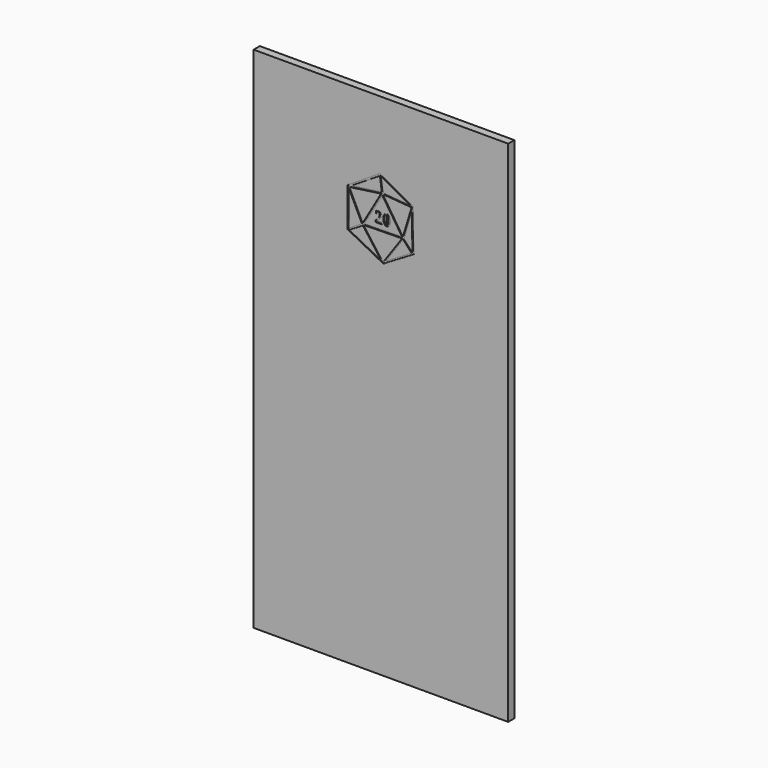
from build123d import *

# Parameters (mm, degrees)
F0_TEXT_SIZE = 10.5298538175
F1_DEPTH     = 4.5
F0_W         = 165
F0_H         = 330
F2_DEPTH     = 5


# Not quite as in the source:
# - Text() gives the source's letters only with a copy of the font that has no kerning and outlines rounded to 1/6400 em; it was checked with that copy


with BuildPart() as f1:
    # F0 (on Front) → F1 (new body)
    with BuildSketch(Plane.XZ):
        Polygon((-14.2118764941, 152.9690027237), (8.9000429127, 140.9807896144), (28.7076475199, 152.7439020574), (28.2208197919, 179.8401356328), (6.6943259021, 191.7312443256), (-14.2118764941, 178.4029453993), align=None)
        Polygon((-4.3210338262, 158.3704430342), (6.9607992757, 143.0644951761), (-13.3234340052, 152.9690027237), align=None, mode=Mode.SUBTRACT)
        Polygon((-5.0023751624, 159.2944927975), (-13.229465754, 154.1256457567), (-13.205724124, 176.2030571699), align=None, mode=Mode.SUBTRACT)
        Polygon((7.4572008215, 180.4599764734), (-4.2189589601, 160.2786725549), (-12.6338905555, 177.6233464479), align=None, mode=Mode.SUBTRACT)
        Polygon((7.8499403882, 181.5359219909), (-11.4866445672, 178.9970174432), (6.6943259021, 190.3372129676), align=None, mode=Mode.SUBTRACT)
        Polygon((21.0209441463, 159.2944927975), (8.9000429127, 142.0140191913), (-3.5439810615, 158.8966995478), align=None, mode=Mode.SUBTRACT)
        Polygon((27.1449846316, 152.9690027237), (10.6374726731, 143.0644951761), (21.7425262656, 158.8966995478), align=None, mode=Mode.SUBTRACT)
        Polygon((21.0209441463, 160.2786725549), (-3.3660947245, 159.8837599158), (8.2897230152, 179.6133667231), align=None, mode=Mode.SUBTRACT)
        Polygon((9.2267788116, 180.4651319981), (27.2039122048, 178.9970174432), (21.6317921941, 160.7204639738), align=None, mode=Mode.SUBTRACT)
        Polygon((27.7245932359, 153.8676992059), (22.3661095936, 159.7770527005), (27.3740378309, 176.2030571699), align=None, mode=Mode.SUBTRACT)
        Polygon((8.9000429127, 181.4443767071), (7.6089858178, 190.2102828026), (26.0070047419, 180.0473252917), align=None, mode=Mode.SUBTRACT)
        with Locations((3.2967818536, 163.0602906743)):
            Text('20', F0_TEXT_SIZE, font='Tinos', font_style=FontStyle.BOLD, text_align=(TextAlign.LEFT, TextAlign.BOTTOM))
    extrude(amount=F1_DEPTH)

    # F0 (on Front) → F2 (join)
    with BuildSketch(Plane.XZ):
        with Locations((7.302631028, 70.7766927429)):
            Rectangle(F0_W, F0_H)
        Polygon((28.7076475199, 152.7439020574), (8.9000429127, 140.9807896144), (-14.2118764941, 152.9690027237), (-14.2118764941, 178.4029453993), (6.6943259021, 191.7312443256), (28.2208197919, 179.8401356328), align=None, mode=Mode.SUBTRACT)
        Polygon((-13.3234340052, 152.9690027237), (6.9607992757, 143.0644951761), (-4.3210338262, 158.3704430342), align=None)
        Polygon((-13.205724124, 176.2030571699), (-13.229465754, 154.1256457567), (-5.0023751624, 159.2944927975), align=None)
        Polygon((-12.6338905555, 177.6233464479), (-4.2189589601, 160.2786725549), (7.4572008215, 180.4599764734), align=None)
        Polygon((6.6943259021, 190.3372129676), (-11.4866445672, 178.9970174432), (7.8499403882, 181.5359219909), align=None)
        Polygon((26.0070047419, 180.0473252917), (7.6089858178, 190.2102828026), (8.9000429127, 181.4443767071), align=None)
        Polygon((21.6317921941, 160.7204639738), (27.2039122048, 178.9970174432), (9.2267788116, 180.4651319981), align=None)
        Polygon((27.3740378309, 176.2030571699), (22.3661095936, 159.7770527005), (27.7245932359, 153.8676992059), align=None)
        Polygon((21.7425262656, 158.8966995478), (10.6374726731, 143.0644951761), (27.1449846316, 152.9690027237), align=None)
        Polygon((-3.5439810615, 158.8966995478), (8.9000429127, 142.0140191913), (21.0209441463, 159.2944927975), align=None)
        Polygon((8.2897230152, 179.6133667231), (-3.3660947245, 159.8837599158), (21.0209441463, 160.2786725549), align=None)
        with BuildLine():
            Line((8.1092541061, 164.2218651736), (8.1092541061, 163.0602906743))
            Line((8.1092541061, 163.0602906743), (3.7393647718, 163.0602906743))
            Line((3.7393647718, 163.0602906743), (3.7393647718, 164.0326568628))
            add(Edge.make_bspline(
                [(3.7393647718, 164.0326568628), (4.1819476901, 164.5048549949), (4.5570737323, 164.8799810372)],
                knots=[0, 0, 0, 1, 1, 1], degree=2))
            add(Edge.make_bspline(
                [(4.5570737323, 164.8799810372), (5.3797185618, 165.6927541287), (5.7597804731, 166.1583711022)],
                knots=[0, 0, 0, 1, 1, 1], degree=2))
            add(Edge.make_bspline(
                [(5.7597804731, 166.1583711022), (6.1398423843, 166.6239880757), (6.3175336674, 167.1225108424)],
                knots=[0, 0, 0, 1, 1, 1], degree=2))
            add(Edge.make_bspline(
                [(6.3175336674, 167.1225108424), (6.4952249506, 167.621033609), (6.4952249506, 168.2577607071)],
                knots=[0, 0, 0, 1, 1, 1], degree=2))
            add(Edge.make_bspline(
                [(6.4952249506, 168.2577607071), (6.4952249506, 168.8188044808), (6.2229295121, 169.1634926643)],
                knots=[0, 0, 0, 1, 1, 1], degree=2))
            add(Edge.make_bspline(
                [(6.2229295121, 169.1634926643), (5.9506340735, 169.5081808479), (5.4981794173, 169.5081808479)],
                knots=[0, 0, 0, 1, 1, 1], degree=2))
            add(Edge.make_bspline(
                [(5.4981794173, 169.5081808479), (5.1789932234, 169.5081808479), (4.9889622678, 169.4415466167)],
                knots=[0, 0, 0, 1, 1, 1], degree=2))
            add(Edge.make_bspline(
                [(4.9889622678, 169.4415466167), (4.7989313122, 169.3749123855), (4.6393382153, 169.2399986335)],
                knots=[0, 0, 0, 1, 1, 1], degree=2))
            Line((4.6393382153, 169.2399986335), (4.4172241113, 168.2429531001))
            Line((4.4172241113, 168.2429531001), (3.9697053241, 168.2429531001))
            Line((3.9697053241, 168.2429531001), (3.9697053241, 169.8109141451))
            add(Edge.make_bspline(
                [(3.9697053241, 169.8109141451), (4.3810277388, 169.903050366), (4.7750746122, 169.9680393076)],
                knots=[0, 0, 0, 1, 1, 1], degree=2))
            add(Edge.make_bspline(
                [(4.7750746122, 169.9680393076), (5.1691214855, 170.0330282491), (5.6314478797, 170.0330282491)],
                knots=[0, 0, 0, 1, 1, 1], degree=2))
            add(Edge.make_bspline(
                [(5.6314478797, 170.0330282491), (6.7666977444, 170.0330282491), (7.371341694, 169.5649433411)],
                knots=[0, 0, 0, 1, 1, 1], degree=2))
            add(Edge.make_bspline(
                [(7.371341694, 169.5649433411), (7.9759856437, 169.0968584331), (7.9759856437, 168.2330813622)],
                knots=[0, 0, 0, 1, 1, 1], degree=2))
            add(Edge.make_bspline(
                [(7.9759856437, 168.2330813622), (7.9759856437, 167.693426354), (7.795826426, 167.2533113702)],
                knots=[0, 0, 0, 1, 1, 1], degree=2))
            add(Edge.make_bspline(
                [(7.795826426, 167.2533113702), (7.6156672084, 166.8131963865), (7.2273788489, 166.3969381027)],
                knots=[0, 0, 0, 1, 1, 1], degree=2))
            add(Edge.make_bspline(
                [(7.2273788489, 166.3969381027), (6.8390904893, 165.980679819), (5.6824518591, 165.0395741341)],
                knots=[0, 0, 0, 1, 1, 1], degree=2))
            add(Edge.make_bspline(
                [(5.6824518591, 165.0395741341), (5.2398689408, 164.6792556988), (4.7265385672, 164.2218651736)],
                knots=[0, 0, 0, 1, 1, 1], degree=2))
            Line((4.7265385672, 164.2218651736), (8.1092541061, 164.2218651736))
        make_face(mode=Mode.SUBTRACT)
        with BuildLine():
            add(Edge.make_bspline(
                [(12.8600279964, 169.1659605988), (13.4251849943, 168.2692777347), (13.4251849943, 166.5367877238)],
                knots=[0, 0, 0, 1, 1, 1], degree=2))
            add(Edge.make_bspline(
                [(13.4251849943, 166.5367877238), (13.4251849943, 162.9566374258), (11.1629117132, 162.9566374258)],
                knots=[0, 0, 0, 1, 1, 1], degree=2))
            add(Edge.make_bspline(
                [(11.1629117132, 162.9566374258), (10.0737299589, 162.9566374258), (9.518444699, 163.872241121)],
                knots=[0, 0, 0, 1, 1, 1], degree=2))
            add(Edge.make_bspline(
                [(9.518444699, 163.872241121), (8.9631594391, 164.7878448163), (8.9631594391, 166.5367877238)],
                knots=[0, 0, 0, 1, 1, 1], degree=2))
            add(Edge.make_bspline(
                [(8.9631594391, 166.5367877238), (8.9631594391, 168.2478889691), (9.518444699, 169.155266216)],
                knots=[0, 0, 0, 1, 1, 1], degree=2))
            add(Edge.make_bspline(
                [(9.518444699, 169.155266216), (10.0737299589, 170.062643463), (11.2040439546, 170.062643463)],
                knots=[0, 0, 0, 1, 1, 1], degree=2))
            add(Edge.make_bspline(
                [(11.2040439546, 170.062643463), (12.2948709985, 170.062643463), (12.8600279964, 169.1659605988)],
                knots=[0, 0, 0, 1, 1, 1], degree=2))
        make_face(mode=Mode.SUBTRACT)
    extrude(amount=F2_DEPTH)


solid = f1.part
